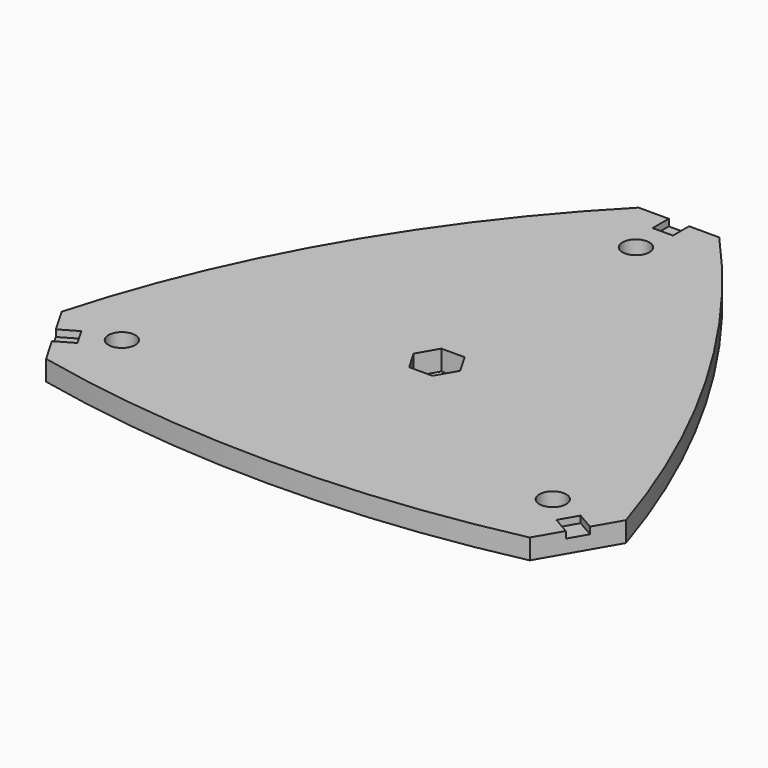
from build123d import *

# Parameters (mm, degrees)
F0_R     = 25.4
F2_DEPTH = 38.1
F0_W     = 38.354
F0_H     = 38.1
F3_DEPTH = 25.4


# Not quite as in the source:
# - a variable given as a bare number and used for a length is read in inches; the dataset says mm whatever the document's units were


with BuildPart() as f2:
    # F0 (on Top) → F2 (new body)
    with BuildSketch(Plane.XY):
        with BuildLine():
            ThreePointArc((-76.2, 571.9231766592), (-355.0918394716, 205.012369106), (-533.4, -219.9704525612))
            Line((-533.4, -219.9704525612), (-504.8885, -269.3538191612))
            Line((-504.8885, -269.3538191612), (-471.8929321158, -250.3038191612))
            Line((-471.8929321158, -250.3038191612), (-452.7159321158, -283.519357498))
            Line((-452.7159321158, -283.519357498), (-485.7115, -302.569357498))
            Line((-485.7115, -302.569357498), (-457.2, -351.952724098))
            ThreePointArc((-457.2, -351.952724098), (0, -401.5140680266), (457.2, -351.952724098))
            Line((457.2, -351.952724098), (485.7115, -302.569357498))
            Line((485.7115, -302.569357498), (452.7159321158, -283.519357498))
            Line((452.7159321158, -283.519357498), (471.8929321158, -250.3038191612))
            Line((471.8929321158, -250.3038191612), (504.8885, -269.3538191612))
            Line((504.8885, -269.3538191612), (533.4, -219.9704525612))
            ThreePointArc((533.4, -219.9704525612), (347.7213828878, 200.7570340133), (76.2, 571.9231766592))
            Line((76.2, 571.9231766592), (19.177, 571.9231766592))
            Line((19.177, 571.9231766592), (19.177, 533.8231766592))
            Line((19.177, 533.8231766592), (-19.177, 533.8231766592))
            Line((-19.177, 533.8231766592), (-19.177, 571.9231766592))
            Line((-19.177, 571.9231766592), (-76.2, 571.9231766592))
        make_face()
        with Locations((-407.3118189755, -235.1615883296)):
            Circle(F0_R, mode=Mode.SUBTRACT)
        Polygon((-21.9970452561, 38.1), (21.9970452561, 38.1), (43.9940905122, 0), (21.9970452561, -38.1), (-21.9970452561, -38.1), (-43.9940905122, 0), align=None, mode=Mode.SUBTRACT)
        with Locations((407.3118189755, -235.1615883296)):
            Circle(F0_R, mode=Mode.SUBTRACT)
        with Locations((0, 470.3231766592)):
            Circle(F0_R, mode=Mode.SUBTRACT)
    extrude(amount=F2_DEPTH)

    # F0 (on Top) → F3 (join)
    with BuildSketch(Plane.XY):
        Polygon((-471.8929321158, -250.3038191612), (-504.8885, -269.3538191612), (-485.7115, -302.569357498), (-452.7159321158, -283.519357498), align=None)
        Polygon((452.7159321158, -283.519357498), (485.7115, -302.569357498), (504.8885, -269.3538191612), (471.8929321158, -250.3038191612), align=None)
        with Locations((0, 552.8731766592)):
            Rectangle(F0_W, F0_H)
    extrude(amount=F3_DEPTH)


solid = f2.part
